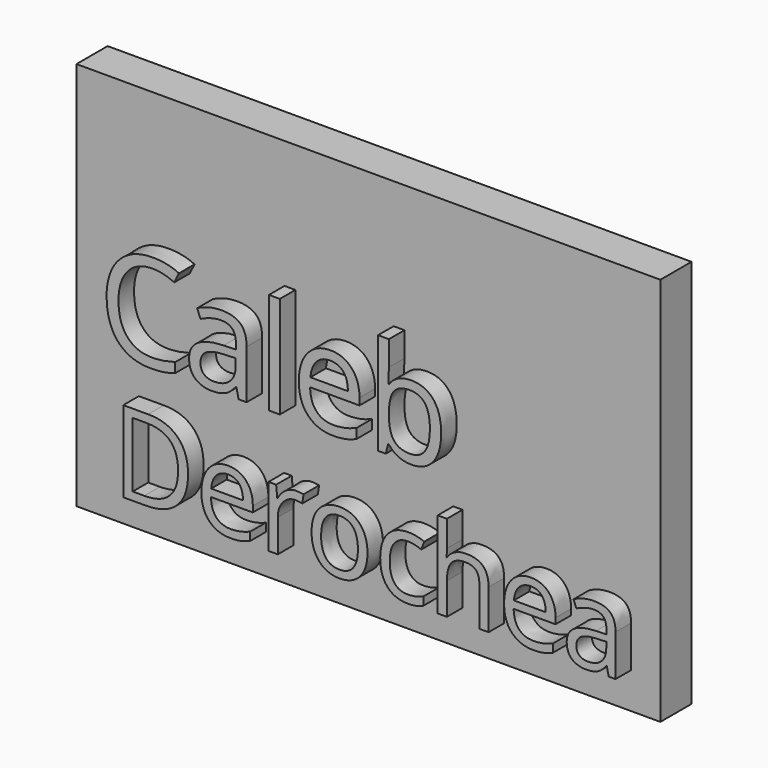
from build123d import *

# Parameters (mm, degrees)
F0_W         = 381
F0_H         = 254
F1_DEPTH     = 12.7
F2_TEXT_SIZE = 87.4140196376
F4_DEPTH     = 12.7
F5_TEXT_SIZE = 74.1658577075
F3_DEPTH     = 12.7


# Not quite as in the source:
# - Text() gives the source's letters only with a copy of the font that has no kerning and outlines rounded to 1/6400 em; it was checked with that copy


with BuildPart() as f1:
    # F0 (on Front) → F1 (new body, symmetric)
    with BuildSketch(Plane.XZ):
        Rectangle(F0_W, F0_H)
    extrude(amount=F1_DEPTH, both=True)

    # F2 (on face) → F4 (join)
    with BuildSketch(Plane.XZ.offset(12.7)):
        with Locations((-166.0212874413, -22.7130055428)):
            Text('Caleb', F2_TEXT_SIZE, font='Open Sans', text_align=(TextAlign.LEFT, TextAlign.BOTTOM))
    extrude(amount=F4_DEPTH)

    # F5 (on face) → F3 (join)
    with BuildSketch(Plane.XZ.offset(12.7)):
        with Locations((-157.075008869, -103.4698039293)):
            Text('Derochea', F5_TEXT_SIZE, font='Open Sans', text_align=(TextAlign.LEFT, TextAlign.BOTTOM))
    extrude(amount=F3_DEPTH)


solid = f1.part
